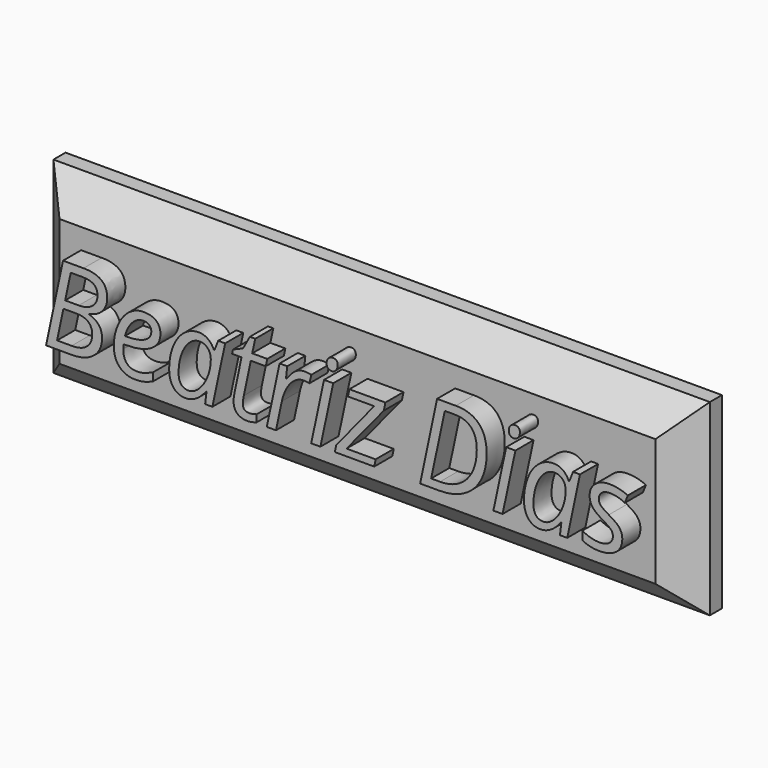
from build123d import *

# Parameters (mm, degrees)
F0_W         = 110.3912852705
F0_H         = 31.5912375227
F1_DEPTH     = 7.62
F2_SIZE      = 5.08
F3_TEXT_SIZE = 18.8680945103
F4_DEPTH     = 3.81


# Not quite as in the source:
# - Text() gives the source's letters only with a copy of the font that has no kerning and outlines rounded to 1/6400 em; it was checked with that copy


with BuildPart() as f1:
    # F0 (on Front) → F1 (new body)
    with BuildSketch(Plane.XZ):
        with Locations((-14.8521605879, 5.6624892168)):
            Rectangle(F0_W, F0_H)
    extrude(amount=F1_DEPTH)

    # F2
    f2_edges = [f1.edges().sort_by_distance(p)[0] for p in [
        (-14.852161, -7.62, 21.458108),
        (-70.047803, -7.62, 5.662489),
        (40.343482, -7.62, 5.662489),
        (-14.852161, -7.62, -10.13313),
    ]]
    chamfer(f2_edges, length=F2_SIZE)

    # F3 (on face) → F4 (join)
    with BuildSketch(Plane.XZ.offset(7.62)):
        with Locations((-64.9678032231, -0.529712881)):
            Text('Beatriz Dias', F3_TEXT_SIZE, font='Open Sans', font_style=FontStyle.ITALIC, text_align=(TextAlign.LEFT, TextAlign.BOTTOM))
    extrude(amount=F4_DEPTH)


solid = f1.part
